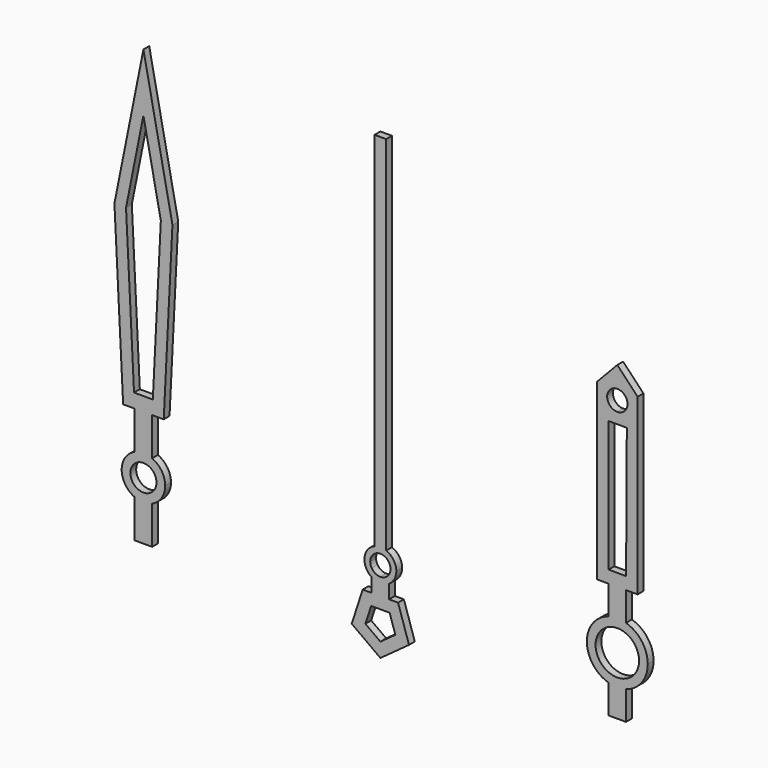
from build123d import *

# Parameters (mm, degrees)
F1_DEPTH = 0.25
F0_W     = 0.3
F0_H     = 0.4009734839
F0_R     = 0.45


# Not quite as in the source:
# - a feature names something its author has since deleted; it is built from what else it names


with BuildPart() as f1:
    # F0 (on Front) → F1 (new body)
    with BuildSketch(Plane.XZ):
        with BuildLine():
            ThreePointArc((-20.5497518182, 1.0062305899), (-21.0916247302, 0.6274950199), (-21.2997518182, 0))
            ThreePointArc((-21.2997518182, 0), (-21.0916247302, -0.6274950199), (-20.5497518182, -1.0062305899))
            ThreePointArc((-20.5497518182, -1.0062305899), (-20.2497518182, -1.05), (-19.9497518182, -1.0062305899))
            ThreePointArc((-19.9497518182, -1.0062305899), (-19.4078789062, -0.6274950199), (-19.1997518182, 0))
            ThreePointArc((-19.1997518182, 0), (-19.4078789062, 0.6274950199), (-19.9497518182, 1.0062305899))
            ThreePointArc((-19.9497518182, 1.0062305899), (-20.2497518182, 1.05), (-20.5497518182, 1.0062305899))
        make_face()
        with BuildLine():
            ThreePointArc((-19.4997518182, 0), (-20.2497518182, -0.75), (-20.9997518182, 0))
            ThreePointArc((-20.9997518182, 0), (-20.2497518182, 0.75), (-19.4997518182, 0))
        make_face(mode=Mode.SUBTRACT)
        with BuildLine():
            Line((-20.5497518182, 2), (-20.5497518182, 1.0062305899))
            ThreePointArc((-20.5497518182, 1.0062305899), (-20.2497518182, 1.05), (-19.9497518182, 1.0062305899))
            Line((-19.9497518182, 1.0062305899), (-19.9497518182, 2))
            Line((-19.9497518182, 2), (-19.9474268439, 2.4239178289))
            Line((-19.9474268439, 2.4239178289), (-20.5497518182, 2.4272212759))
            Line((-20.5497518182, 2.4272212759), (-20.5497518182, 2))
        make_face()
        with BuildLine():
            ThreePointArc((-19.9497518182, -1.0062305899), (-20.2497518182, -1.05), (-20.5497518182, -1.0062305899))
            Line((-20.5497518182, -1.0062305899), (-20.5497518182, -2))
            Line((-20.5497518182, -2), (-19.9497518182, -2))
            Line((-19.9497518182, -2), (-19.9497518182, -1.0062305899))
        make_face()
        with BuildLine():
            Line((-20.9497518182, 2), (-20.5497518182, 2))
            Line((-20.5497518182, 2), (-20.5497518182, 2.4272212759))
            Line((-20.5497518182, 2.4272212759), (-20.5497518182, 6.936291784))
            Line((-20.5497518182, 6.936291784), (-20.2497518182, 6.936291784))
            Line((-20.2497518182, 6.936291784), (-20.2497518182, 7.3125319198))
            ThreePointArc((-20.2497518182, 7.3125319198), (-20.5997518182, 7.6625319198), (-20.2497518182, 8.0125319198))
            Line((-20.2497518182, 8.0125319198), (-20.2497518182, 8.7373927236))
            Line((-20.2497518182, 8.7373927236), (-20.9497518182, 8))
            Line((-20.9497518182, 8), (-20.9497518182, 2))
        make_face()
        with BuildLine():
            Line((-19.9474268439, 2.4239178289), (-19.9497518182, 2))
            Line((-19.9497518182, 2), (-19.5497518182, 2))
            Line((-19.5497518182, 2), (-19.5497518182, 8))
            Line((-19.5497518182, 8), (-20.2497518182, 8.7373927236))
            Line((-20.2497518182, 8.7373927236), (-20.2497518182, 8.0125319198))
            ThreePointArc((-20.2497518182, 8.0125319198), (-20.0022644448, 7.9100192932), (-19.8997518182, 7.6625319198))
            ThreePointArc((-19.8997518182, 7.6625319198), (-20.0022644448, 7.4150445464), (-20.2497518182, 7.3125319198))
            Line((-20.2497518182, 7.3125319198), (-20.2497518182, 6.936291784))
            Line((-20.2497518182, 6.936291784), (-19.9226787618, 6.936291784))
            Line((-19.9226787618, 6.936291784), (-19.9474268439, 2.4239178289))
        make_face()
    extrude(amount=F1_DEPTH)


with BuildPart() as f1b:
    # F0 (on Front) → F1, piece 2 (new body)
    with BuildSketch(Plane.XZ):
        with BuildLine():
            ThreePointArc((-28.6187018186, 0.5123475383), (-28.8728493717, 0.3102418412), (-28.9687018186, 0))
            Line((-28.9687018186, 0), (-28.7687018186, 0))
            ThreePointArc((-28.7687018186, 0), (-28.7289436597, 0.1620185175), (-28.6187018186, 0.2872281323))
            Line((-28.6187018186, 0.2872281323), (-28.6187018186, 0.5123475383))
        make_face()
        with BuildLine():
            Line((-28.7687018186, 0), (-28.9687018186, 0))
            ThreePointArc((-28.9687018186, 0), (-28.9021788087, -0.262202212), (-28.7187018186, -0.4609772229))
            Line((-28.7187018186, -0.4609772229), (-28.7187018186, -0.1802775638))
            ThreePointArc((-28.7187018186, -0.1802775638), (-28.7559702577, -0.0935414347), (-28.7687018186, 0))
        make_face()
        with BuildLine():
            Line((-28.6187018186, 13), (-28.6187018186, 0.5123475383))
            ThreePointArc((-28.6187018186, 0.5123475383), (-28.4187018186, 0.55), (-28.2187018186, 0.5123475383))
            Line((-28.2187018186, 0.5123475383), (-28.2187018186, 13))
            Line((-28.2187018186, 13), (-28.6187018186, 13))
        make_face()
        with BuildLine():
            ThreePointArc((-28.2187018186, 0.5123475383), (-28.4187018186, 0.55), (-28.6187018186, 0.5123475383))
            Line((-28.6187018186, 0.5123475383), (-28.6187018186, 0.2872281323))
            ThreePointArc((-28.6187018186, 0.2872281323), (-28.4187018186, 0.35), (-28.2187018186, 0.2872281323))
            Line((-28.2187018186, 0.2872281323), (-28.2187018186, 0.5123475383))
        make_face()
        with BuildLine():
            Line((-28.7187018186, -0.1802775638), (-28.7187018186, -0.4609772229))
            ThreePointArc((-28.7187018186, -0.4609772229), (-28.5751667147, -0.5272748205), (-28.4187018186, -0.55))
            Line((-28.4187018186, -0.55), (-28.4187018186, -0.35))
            ThreePointArc((-28.4187018186, -0.35), (-28.5910428362, -0.3046285831), (-28.7187018186, -0.1802775638))
        make_face()
        with BuildLine():
            ThreePointArc((-28.4187018186, -0.55), (-28.5751667147, -0.5272748205), (-28.7187018186, -0.4609772229))
            Line((-28.7187018186, -0.4609772229), (-28.7187018186, -0.9359067772))
            Line((-28.7187018186, -0.9359067772), (-28.4187018186, -0.9359067772))
            Line((-28.4187018186, -0.9359067772), (-28.4187018186, -0.55))
        make_face()
        with BuildLine():
            ThreePointArc((-27.8687018186, 0), (-27.9645542655, 0.3102418411), (-28.2187018186, 0.5123475383))
            Line((-28.2187018186, 0.5123475383), (-28.2187018186, 0.2872281323))
            ThreePointArc((-28.2187018186, 0.2872281323), (-28.1084599774, 0.1620185175), (-28.0687018186, 0))
            Line((-28.0687018186, 0), (-27.8687018186, 0))
        make_face()
        with BuildLine():
            Line((-28.4187018186, -0.35), (-28.4187018186, -0.55))
            ThreePointArc((-28.4187018186, -0.55), (-28.2622369225, -0.5272748205), (-28.1187018186, -0.4609772229))
            Line((-28.1187018186, -0.4609772229), (-28.1187018186, -0.1802775638))
            ThreePointArc((-28.1187018186, -0.1802775638), (-28.246360801, -0.3046285831), (-28.4187018186, -0.35))
        make_face()
        with BuildLine():
            ThreePointArc((-28.1187018186, -0.4609772229), (-28.2622369225, -0.5272748205), (-28.4187018186, -0.55))
            Line((-28.4187018186, -0.55), (-28.4187018186, -0.9359067772))
            Line((-28.4187018186, -0.9359067772), (-28.1187018186, -0.9359067772))
            Line((-28.1187018186, -0.9359067772), (-28.1187018186, -0.4609772229))
        make_face()
        with Locations((-28.5687018186, -1.1363935191)):
            Rectangle(F0_W, F0_H)
        Polygon((-28.7187018186, -1.3368802611), (-28.7187018186, -0.9359067772), (-29.0288436917, -0.9359067772), (-29.4059321072, -2.0964655857), (-28.4187018186, -2.8137303753), (-28.4187018186, -2.318099892), (-28.9345595064, -1.9433073434), (-28.737519403, -1.3368802611), align=None)
        with BuildLine():
            ThreePointArc((-28.1187018186, -0.4609772229), (-27.9352248284, -0.262202212), (-27.8687018186, 0))
            Line((-27.8687018186, 0), (-28.0687018186, 0))
            ThreePointArc((-28.0687018186, 0), (-28.0814333795, -0.0935414347), (-28.1187018186, -0.1802775638))
            Line((-28.1187018186, -0.1802775638), (-28.1187018186, -0.4609772229))
        make_face()
        with Locations((-28.2687018186, -1.1363935191)):
            Rectangle(F0_W, F0_H)
        Polygon((-27.8085599455, -0.9359067772), (-28.1187018186, -0.9359067772), (-28.1187018186, -1.3368802611), (-28.0998842342, -1.3368802611), (-27.9028441308, -1.9433073434), (-28.4187018186, -2.318099892), (-28.4187018186, -2.8137303753), (-27.43147153, -2.0964655857), align=None)
    extrude(amount=F1_DEPTH)


with BuildPart() as f1c:
    # F0 (on Front) → F1, piece 3 (new body)
    with BuildSketch(Plane.XZ):
        Polygon((-35.587651819, 8), (-36.587651819, 13), (-37.587651819, 8), (-37.287651819, 2), (-36.887651819, 2), (-36.9116376011, 2.4797156414), (-37.187651819, 8), (-36.587651819, 11), (-35.987651819, 8), (-36.2636660369, 2.4797156414), (-36.287651819, 2), (-35.887651819, 2), align=None)
        with BuildLine():
            Line((-36.287651819, 0.6873863542), (-36.287651819, 2))
            Line((-36.287651819, 2), (-36.887651819, 2))
            Line((-36.887651819, 2), (-36.887651819, 0.6873863542))
            ThreePointArc((-36.887651819, 0.6873863542), (-36.587651819, 0.75), (-36.287651819, 0.6873863542))
        make_face()
        Polygon((-36.887651819, 2), (-36.287651819, 2), (-36.2636660369, 2.4797156414), (-36.9116376011, 2.4797156414), align=None)
        with BuildLine():
            ThreePointArc((-35.837651819, 0), (-35.9601567991, 0.4107919181), (-36.287651819, 0.6873863542))
            ThreePointArc((-36.287651819, 0.6873863542), (-36.587651819, 0.75), (-36.887651819, 0.6873863542))
            ThreePointArc((-36.887651819, 0.6873863542), (-37.337651819, 0), (-36.887651819, -0.6873863542))
            ThreePointArc((-36.887651819, -0.6873863542), (-36.587651819, -0.75), (-36.287651819, -0.6873863542))
            ThreePointArc((-36.287651819, -0.6873863542), (-35.9601567991, -0.4107919181), (-35.837651819, 0))
        make_face()
        with Locations((-36.587651819, 0)):
            Circle(F0_R, mode=Mode.SUBTRACT)
        with BuildLine():
            ThreePointArc((-36.287651819, -0.6873863542), (-36.587651819, -0.75), (-36.887651819, -0.6873863542))
            Line((-36.887651819, -0.6873863542), (-36.887651819, -2))
            Line((-36.887651819, -2), (-36.287651819, -2))
            Line((-36.287651819, -2), (-36.287651819, -0.6873863542))
        make_face()
    extrude(amount=F1_DEPTH)


solid = Compound([f1.part, f1b.part, f1c.part])
